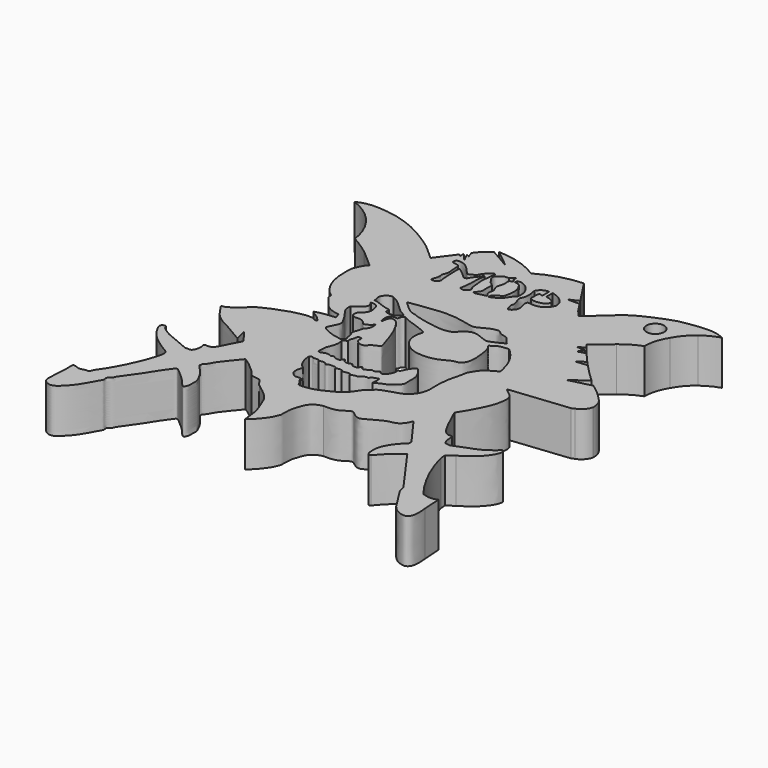
from build123d import *

# Parameters (mm, degrees)
F1_DEPTH = 5
F2_D     = 2
F2_DEPTH = 13.5
F2_TIP   = 0.600860619


with BuildPart() as f1:
    # F0 (on Top) → F1 (new body)
    with BuildSketch(Plane.XY):
        with BuildLine():
            ThreePointArc((-20.6029620022, 21.1226996034), (-17.5915636948, 19.019722507), (-16.1475036293, 15.6424865127))
            ThreePointArc((-16.1475036293, 15.6424865127), (-15.0464363703, 14.9775310986), (-13.9912227169, 14.2419775948))
            Line((-13.9912227169, 14.2419775948), (-11.9417123497, 12.4597940594))
            add(Edge.make_bspline(
                [(-12.1965548024, 7.2102304548), (-12.3502998605, 7.4831671233), (-12.5147308437, 7.918563535), (-12.7293340893, 8.6338874307), (-12.8327536648, 9.5869088664), (-12.8349054333, 10.6792935822), (-12.8027446008, 11.1125926196), (-12.2509882508, 12.2447047975), (-12.0226823195, 12.4034826204), (-11.9417123497, 12.4597940594)],
                knots=[0.8610480247, 0.8610480247, 0.8610480247, 0.8610480247, 0.8811330773, 0.9001834199, 0.9227784911, 0.945893675, 0.9616042621, 0.9863827378, 1, 1, 1, 1], degree=3))
            Line((-12.1965548024, 7.2102304548), (-11.8690758114, 6.7050356711))
            add(Edge.make_bspline(
                [(-11.6388598274, 6.4153944981), (-11.7173747261, 6.5058097894), (-11.7950645675, 6.6040888756), (-11.8690758114, 6.7050356711)],
                knots=[0.8422887794, 0.8422887794, 0.8422887794, 0.8422887794, 0.8493024804, 0.8493024804, 0.8493024804, 0.8493024804], degree=3))
            Line((-11.6388598274, 6.4153944981), (-11.4010572433, 6.1705708504))
            add(Edge.make_bspline(
                [(-8.2604521886, 3.4468797967), (-8.4593902999, 3.4581469309), (-8.8945130912, 3.5751560394), (-9.4160163716, 3.7356827733), (-9.9909022798, 4.1606108445), (-10.1208112278, 4.4103187237), (-10.540425506, 4.8665439074), (-10.7332609152, 5.1282105819), (-11.0928393262, 5.6046851275), (-10.9504645183, 5.8646077471), (-11.2233401518, 6.0114178789), (-11.4010572433, 6.1705708504)],
                knots=[0.6950364261, 0.6950364261, 0.6950364261, 0.6950364261, 0.7129994084, 0.7302227681, 0.7486757288, 0.761065719, 0.7782452685, 0.7921804993, 0.8088061225, 0.8190631278, 0.835195334, 0.835195334, 0.835195334, 0.835195334], degree=3))
            add(Edge.make_bspline(
                [(-8.04425776, 2.8521639761), (-7.9018632901, 2.858641559), (-7.7057651467, 2.8469124875), (-7.5831119329, 2.8591957281), (-7.4479762519, 2.8711507591), (-7.505413234, 3.0021417322), (-7.7961410323, 3.4541077042), (-7.9021987786, 3.4673998991), (-8.1104128522, 3.438382112), (-8.2604521886, 3.4468797967)],
                knots=[0.6221073953, 0.6221073953, 0.6221073953, 0.6221073953, 0.6354090806, 0.6434381095, 0.6504907803, 0.6579034221, 0.674423125, 0.6814887257, 0.6950364261, 0.6950364261, 0.6950364261, 0.6950364261], degree=3))
            add(Edge.make_bspline(
                [(-12.3581970111, -5.6642671116), (-12.5904511424, -5.5812313985), (-13.0193487189, -5.3035516251), (-13.6976748576, -4.9215909797), (-14.6685644807, -4.3370329977), (-15.1784801551, -4.1175978961), (-15.7822788069, -3.7457351464), (-16.4224422592, -3.1712375943), (-16.7599481469, -2.645328985), (-17.0923394133, -2.2265555734), (-17.2212769529, -2.0106109394), (-17.3896610291, -1.7573138007), (-17.1319935898, -1.7444644607), (-16.9508920629, -1.7170211764), (-16.347646044, -1.3596815627), (-15.645035849, -0.848528458), (-15.2656555451, -0.37634208), (-15.0754605235, -0.2604548851), (-14.734679896, 0.0366996912), (-14.178640127, 0.2610233151), (-13.6015369056, 0.5853071698), (-12.8447573829, 0.8220084278), (-12.1648413666, 1.1160641981), (-11.595046482, 1.272849878), (-10.9995895136, 1.4056237292), (-10.3895434203, 1.5428319889), (-9.6396418204, 1.5312353279), (-9.4289246698, 1.417578834), (-9.3011799222, 1.2945856497), (-8.942384529, 1.276901966), (-9.0026734788, 1.4242730407), (-9.167712209, 1.5846567137), (-9.5309989371, 1.9880562353), (-10.2229826163, 2.3564941518), (-10.2892403261, 2.4314994287), (-10.302815711, 2.5023911971), (-10.2349771538, 2.5157399501), (-10.1672388489, 2.5081225633), (-9.8508510482, 2.6248918916), (-9.3754645701, 2.724901108), (-8.7177845236, 2.771494927), (-8.242723901, 2.8431356698), (-8.04425776, 2.8521639761)],
                knots=[0.0199809931, 0.0199809931, 0.0199809931, 0.0199809931, 0.0393496026, 0.0597271396, 0.0835928224, 0.1005434587, 0.1193240265, 0.1403089769, 0.158438488, 0.174595577, 0.1865174997, 0.1969260736, 0.2062553482, 0.2161564821, 0.2346403213, 0.2565308226, 0.2735861318, 0.2840287475, 0.2987882298, 0.3163830901, 0.3348196829, 0.3549968985, 0.3744741565, 0.3917947559, 0.4092021997, 0.4275883294, 0.4468781727, 0.4573928431, 0.4670857793, 0.4791440786, 0.4858131114, 0.4964248036, 0.5137198846, 0.5335221874, 0.5402661667, 0.54539731, 0.5505805585, 0.5563736505, 0.5689626198, 0.5850282163, 0.603567812, 0.6221073953, 0.6221073953, 0.6221073953, 0.6221073953], degree=3))
            Line((-12.3581970111, -5.6642671116), (-12.6814246178, -4.32879664))
            Line((-12.6814246178, -4.32879664), (-11.5899201483, -5.809974391))
            add(Edge.make_bspline(
                [(-11.5899201483, -5.809974391), (-11.761671997, -6.1515096125), (-12.1023394972, -6.8289401669), (-12.5988375731, -7.7793439457), (-13.0560319176, -8.6202165569), (-14.0611028159, -8.3810100434), (-13.6893610625, -9.0087176513), (-14.0412955656, -10.064201964), (-14.4145629084, -9.9866002857), (-14.6357854762, -9.9824532437), (-14.8157372232, -10.0789508645), (-16.281058055, -9.3570080841), (-16.8233033734, -9.212552149), (-17.7368272991, -8.7952962439), (-18.6917469793, -8.1412114636), (-18.6420124904, -7.8298569891), (-18.9893398137, -7.7692027771), (-19.3106699916, -8.0342693106), (-19.0208951386, -8.680301289), (-18.5961106249, -9.4212285605), (-17.9192155256, -10.1285007663), (-16.9946139375, -10.8428939411), (-16.0873411982, -11.4169768576), (-15.5695893324, -11.6777704888), (-15.5798054281, -12.459245462), (-16.2005580806, -14.2818357649), (-17.0898354691, -16.1841050865), (-17.9990009864, -17.7647021784), (-18.4788322489, -18.2943472783), (-18.6390866322, -18.8999775429), (-19.0640131121, -18.7354536271), (-19.615346749, -19.099336736), (-20.4150388035, -18.6117409365), (-20.5369505302, -18.9048172824), (-20.4745198098, -19.3549123287), (-20.5633095325, -20.6757675795), (-20.6104330874, -21.6089482824), (-20.6526211227, -22.2395843559), (-20.5013571763, -22.6079781881), (-20.1803826553, -22.8383312321), (-19.7318715009, -23.0137189608), (-19.2193538265, -22.8744691129), (-18.7003457403, -22.3844825927), (-18.0593824453, -21.7304410154), (-17.3644822048, -20.6360646539), (-16.8172253424, -19.5595324477), (-16.5714630416, -19.2353425016), (-16.7570703992, -18.7742146415), (-16.2597684066, -18.5543558491), (-16.1987565932, -18.1739453761), (-15.4476121444, -17.1851846193), (-14.4609757351, -15.7871082425), (-13.8660241761, -14.7528565805), (-13.1529493933, -13.8016805992), (-12.8956471778, -13.4382777026), (-12.1402183108, -14.1250996886), (-11.3282640309, -14.7873756688), (-10.5542045699, -15.7471405416), (-10.4835155205, -15.8130234223), (-10.2753596318, -15.9090116166), (-10.1982709972, -15.7072660935), (-10.0523513853, -15.47296592), (-10.0750379365, -14.8415342807), (-10.0095114609, -14.292303092), (-10.5072174977, -13.352197784), (-10.9709437469, -12.6407861923), (-11.750335269, -11.9121516462), (-11.7388578236, -11.78510289), (-11.6600968913, -11.6740233806), (-11.7464815118, -11.5146223585), (-11.3969134992, -11.2917363839), (-11.0903574926, -10.5436660123), (-10.3206257246, -9.6014779347), (-9.6643011605, -8.7958952944), (-9.313037619, -8.364749141)],
                knots=[0, 0, 0, 0, 0.0179813568, 0.0356657813, 0.051329078, 0.0651099748, 0.0766372495, 0.0935148294, 0.1026170722, 0.1101464218, 0.1172045658, 0.1380930678, 0.1517065559, 0.1686436507, 0.1862776399, 0.1941540818, 0.2029227342, 0.2124825546, 0.225756734, 0.2415613643, 0.2581194594, 0.2765443366, 0.2940493854, 0.305875686, 0.3193973265, 0.3426850978, 0.3679383695, 0.3903240637, 0.4046447144, 0.416373877, 0.4260507347, 0.4393671317, 0.4542499545, 0.4614022989, 0.4726186512, 0.4920540368, 0.5088224874, 0.5218416547, 0.5320047128, 0.5423752, 0.5538059057, 0.5656121747, 0.5796000293, 0.5956835108, 0.6152465419, 0.6336595403, 0.6438739959, 0.6542959706, 0.6653348002, 0.6752500928, 0.6936720731, 0.7160143125, 0.7349445332, 0.7530770661, 0.7623269307, 0.7776086779, 0.7964830854, 0.8143398494, 0.8197448066, 0.8267371939, 0.8336105298, 0.8424634875, 0.8555147647, 0.8681538827, 0.8849009963, 0.9015710239, 0.9181986098, 0.9233461612, 0.9291090514, 0.9352376166, 0.9449772073, 0.9599565939, 0.9785688524, 1, 1, 1, 1], degree=3))
            add(Edge.make_bspline(
                [(-2.1674414165, -17.3634011298), (-2.2083754085, -17.0670616618), (-2.2889277013, -16.483907601), (-2.3687674967, -15.6105740644), (-2.5056489877, -15.180468512), (-2.7149333593, -14.5715948025), (-3.0057117915, -13.9808265561), (-3.2610484039, -13.1945992574), (-4.0167638414, -12.4073570072), (-4.8092463789, -11.8571987969), (-5.5319002932, -11.302861115), (-5.811512679, -10.4873353187), (-7.0168671674, -10.6046346662), (-7.2475569156, -9.9817356818), (-7.8224846209, -9.4881864383), (-8.3692761757, -9.0207724304), (-8.9599333798, -8.5668206068), (-9.2080848604, -8.4248106056), (-9.313037619, -8.364749141)],
                knots=[0, 0, 0, 0, 0.0689009641, 0.1355873292, 0.1841509068, 0.2409673149, 0.2997760241, 0.3648024212, 0.4395050627, 0.5112588235, 0.5792603578, 0.641576026, 0.7135666611, 0.7681324686, 0.8301936499, 0.8927655608, 0.9546464515, 1, 1, 1, 1], degree=3))
            add(Edge.make_bspline(
                [(1.6768131172, -11.058810167), (1.4498258422, -11.1119512781), (0.9778327854, -11.2224519019), (0.3269774066, -11.7855546665), (0.0646584188, -12.5740691446), (-0.1527713728, -13.1811284517), (-0.2097492346, -13.8412703608), (-0.2329829382, -14.3559228246), (-0.1924124239, -14.7284014532), (-0.3964332077, -15.1432360242), (-0.5584881611, -15.5322147196), (-0.8834596458, -15.9997141654), (-1.136769425, -16.3273670151), (-1.4494183058, -16.7034452851), (-1.7552805529, -17.0057514481), (-2.0248897803, -17.2397029532), (-2.1674414165, -17.3634011298)],
                knots=[0, 0, 0, 0, 0.0808085825, 0.1680318417, 0.255018001, 0.3325718365, 0.4106102442, 0.4794380848, 0.5373322163, 0.601038936, 0.6646014985, 0.736379439, 0.799216676, 0.8654979694, 0.928884168, 1, 1, 1, 1], degree=3))
            add(Edge.make_bspline(
                [(9.6936440095, -8.3805257455), (9.6053730454, -8.6062045499), (9.4248404792, -9.0677648615), (8.7644476462, -9.7019868071), (7.8391484374, -9.6802752734), (5.9960176715, -10.8377393732), (5.5709076534, -10.9653133541), (5.084651123, -10.8502179729), (4.5962398094, -10.4018320652), (4.31685127, -10.2638895059), (3.9607013957, -10.3984297753), (3.3525593133, -10.8740414946), (2.5884025531, -11.0445659428), (2.1036380444, -11.0617450847), (1.815664393, -11.059764931), (1.6768131172, -11.058810167)],
                knots=[0, 0, 0, 0, 0.0813790915, 0.1664372465, 0.2589445345, 0.3967526344, 0.4592648623, 0.5231293603, 0.6003716548, 0.6506866848, 0.7055950558, 0.7891929021, 0.8731143432, 0.9388199746, 1, 1, 1, 1], degree=3))
            Line((9.6936440095, -8.3805257455), (12.0183676481, -11.5794716403))
            Line((12.0183676481, -11.5794716403), (12.0183676481, -11.9077553973))
            add(Edge.make_bspline(
                [(10.380987078, -15.4800917953), (10.3387332997, -15.117733548), (10.246426762, -14.3261348663), (11.0215378886, -12.8784303298), (11.6925110223, -12.2250621944), (12.0183676481, -11.9077553973)],
                knots=[0, 0, 0, 0, 0.3027512141, 0.6613826615, 1, 1, 1, 1], degree=3))
            add(Edge.make_bspline(
                [(10.8141666278, -15.8001016825), (10.7427231899, -15.8416310013), (10.5683574389, -15.9429879778), (10.4505342148, -15.6519071454), (10.380987078, -15.4800917953)],
                knots=[0, 0, 0, 0, 0.4097332049, 1, 1, 1, 1], degree=3))
            add(Edge.make_bspline(
                [(13.1668290123, -13.602392748), (12.7702129139, -13.8888540012), (11.9451949477, -14.4847342025), (11.2007367392, -15.350526951), (10.8141666278, -15.8001016825)],
                knots=[0, 0, 0, 0, 0.4807363168, 1, 1, 1, 1], degree=3))
            Line((13.1668290123, -13.602392748), (16.9230792671, -18.8517868519))
            add(Edge.make_bspline(
                [(17.1615090221, -19.6730475873), (17.034785822, -19.4525867701), (16.9331803918, -19.186956808), (16.9230792671, -18.8517868519)],
                knots=[0, 0, 0, 0, 0.8551712949, 0.8551712949, 0.8551712949, 0.8551712949], degree=3))
            Line((17.1615090221, -19.6730475873), (18.6557825655, -22.0313183963))
            add(Edge.make_bspline(
                [(20.9009312093, -20.7379574093), (20.946669412, -21.0068443415), (21.0667752252, -22.424045845), (20.5441691625, -22.9480911155), (20.0814156096, -23.008898701), (19.1827038868, -22.6588555056), (18.8077084078, -22.2142964537), (18.6557825655, -22.0313183963)],
                knots=[0, 0, 0, 0, 0.2759456386, 0.4545875307, 0.5943096845, 0.8039768536, 1, 1, 1, 1], degree=3))
            Line((20.9009312093, -20.7379574093), (20.7737311721, -18.7153462321))
            add(Edge.make_bspline(
                [(19.0693489557, -18.7153462321), (19.3211115884, -18.7936733033), (19.916140688, -18.9445847276), (20.3488546888, -18.8852960675), (20.7737311721, -18.7153462321)],
                knots=[0, 0, 0, 0, 0.4817386314, 1, 1, 1, 1], degree=3))
            ThreePointArc((19.0693489557, -18.7153462321), (17.1945449581, -15.6929535506), (15.9742087126, -12.3522160575))
            Line((15.9742087126, -12.3522160575), (15.9212257713, -11.7296464741))
            Line((15.9212257713, -11.7296464741), (16.7331937701, -11.1593846232))
            add(Edge.make_bspline(
                [(19.5059552789, -8.0829588094), (19.4447040558, -8.5108317435), (19.076332208, -9.2460772627), (17.9914928687, -10.3808130068), (17.1422320797, -10.9105939373), (16.7331937701, -11.1593846232)],
                knots=[0, 0, 0, 0, 0.310219277, 0.6584804582, 1, 1, 1, 1], degree=3))
            ThreePointArc((19.5059552789, -8.0829588094), (19.2350807313, -7.7977856695), (18.9642061838, -8.0829588094))
            add(Edge.make_bspline(
                [(15.0774473823, -9.967437324), (16.5505504071, -9.4062854741), (17.5287417336, -9.0468549853), (18.2133857161, -8.660803549), (18.9642061838, -8.0829588094)],
                knots=[0, 0, 0, 0, 0.5565007534, 1, 1, 1, 1], degree=3))
            Line((15.0774473823, -9.967437324), (14.5304155103, -9.8842515916))
            add(Edge.make_bspline(
                [(11.4801516756, -4.8446576111), (12.2792130652, -6.6117397342), (13.2242516061, -8.8699425893), (14.4148425893, -8.2242481179), (14.1074610189, -9.4350335972), (14.5304155103, -9.8842515916)],
                knots=[0, 0, 0, 0, 0.5155027122, 0.7007845535, 1, 1, 1, 1], degree=3))
            add(Edge.make_bspline(
                [(12.2916540131, 1.5507938806), (12.7276787534, 1.0922398651), (13.6267942877, 0.793434585), (13.4155968414, -1.2858010843), (12.7945104614, -2.7060380671), (11.4801516756, -4.8446576111)],
                knots=[0, 0, 0, 0, 0.2667013683, 0.5335681874, 1, 1, 1, 1], degree=3))
            Line((12.2916540131, 1.5507938806), (18.9940966666, 2.2610761225))
            Line((18.9940966666, 2.2610761225), (19.305286929, 2.4047526531))
            ThreePointArc((19.305286929, 2.4047526531), (20.0097990037, 2.8651506455), (20.4079579562, 3.6066174507))
            ThreePointArc((20.4079579562, 3.6066174507), (20.3193874403, 4.3080407583), (19.9958346784, 4.9366527237))
            ThreePointArc((19.9958346784, 4.9366527237), (18.9806691644, 5.9619052319), (17.8415514529, 6.8474076688))
            Line((17.8415514529, 6.8474076688), (15.2579825372, 6.2031652778))
            Line((15.2579825372, 6.2031652778), (17.1197786733, 7.4977375506))
            ThreePointArc((17.1197786733, 7.4977375506), (16.0491412163, 8.5243825489), (15.0177698901, 9.5904677728))
            Line((15.0177698901, 9.5904677728), (13.6827398092, 9.4481641427))
            Line((13.6827398092, 9.4481641427), (14.5777972838, 10.0705290551))
            ThreePointArc((14.5777972838, 10.0705290551), (14.0339347858, 10.6866031408), (13.5029950802, 11.3138484875))
            Line((13.5029950802, 11.3138484875), (12.5840436667, 11.0233156011))
            Line((12.5840436667, 11.0233156011), (13.0566162989, 11.6376606748))
            Line((13.0566162989, 11.6376606748), (12.4895293266, 11.4643834531))
            Line((12.4895293266, 11.4643834531), (12.8675876185, 11.763679795))
            Line((12.8675876185, 11.763679795), (12.0799662545, 11.7006702349))
            Line((12.0799662545, 11.7006702349), (12.8092804911, 12.1751222925))
            ThreePointArc((12.8092804911, 12.1751222925), (12.6443146642, 12.3873848258), (12.4807959896, 12.6007641829))
            Line((12.4807959896, 12.6007641829), (14.5000191405, 14.3246697262))
            ThreePointArc((14.5000191405, 14.3246697262), (15.5107148946, 15.0425023951), (16.6326500475, 15.5698079616))
            ThreePointArc((16.6326500475, 15.5698079616), (16.8245383582, 16.9374935756), (17.400925979, 18.1925483048))
            ThreePointArc((17.400925979, 18.1925483048), (18.1163270549, 19.25582228), (19.0566964447, 20.1264861971))
            ThreePointArc((19.0566964448, 20.1264861971), (19.9676202839, 20.6998781196), (20.9641419351, 21.1067013443))
            ThreePointArc((20.9641419351, 21.1067013443), (20.0622769035, 21.4273714063), (19.1106745535, 21.5305353114))
            ThreePointArc((19.1106745535, 21.5305353114), (17.494918218, 21.3939271519), (15.8990386297, 21.1067013443))
            ThreePointArc((15.8990386297, 21.1067013443), (14.2592549209, 20.5084373442), (12.6720489934, 19.7820849716))
            ThreePointArc((12.6720489934, 19.7820849716), (11.8479697713, 19.298407767), (11.0957566649, 18.7091492116))
            Line((11.0957566649, 18.7091492116), (8.5127558559, 16.3910705596))
            Line((8.5127558559, 16.3910705596), (7.823956199, 17.2255784273))
            Line((7.823956199, 17.2255784273), (7.1296900244, 18.291907385))
            Line((7.1296900244, 18.291907385), (5.743692629, 18.291907385))
            Line((5.743692629, 18.291907385), (6.8139770912, 18.7768133983))
            Line((6.8139770912, 18.7768133983), (4.9760327674, 21.5997267514))
            ThreePointArc((4.9760327674, 21.5997267514), (2.470754193, 21.1792888514), (0.1411859703, 20.1662238687))
            ThreePointArc((0.1411859703, 20.1662238687), (-2.1388945551, 21.2114676219), (-4.6169091947, 21.5997267514))
            Line((-4.6169091947, 21.5997267514), (-2.5629734155, 19.9449639767))
            Line((-2.5629734155, 19.9449639767), (-4.9981252836, 21.3476927034))
            ThreePointArc((-4.9981252836, 21.3476927034), (-5.7618963683, 20.7054799466), (-6.4152670093, 19.9512317777))
            Line((-6.4152670093, 19.9512317777), (-6.1913165264, 19.281739369))
            Line((-6.1913165264, 19.281739369), (-6.5142409876, 19.3998813629))
            Line((-6.5142409876, 19.3998813629), (-6.0180397704, 18.4389837086))
            Line((-6.0180397704, 18.4389837086), (-6.8394649689, 19.3754563593))
            Line((-6.8394649689, 19.3754563593), (-6.8394649689, 18.8564229756))
            Line((-6.8394649689, 18.8564229756), (-7.0873237208, 19.0390309396))
            Line((-7.0873237208, 19.0390309396), (-8.6397584528, 16.9318690896))
            Line((-8.6397584528, 16.9318690896), (-10.2622583508, 18.3810908347))
            ThreePointArc((-10.2622583508, 18.3810908347), (-11.3785350691, 19.1686702966), (-12.5463595614, 19.8775716126))
            ThreePointArc((-12.5463595614, 19.8775716126), (-15.3498488558, 21.1074830333), (-18.3747559786, 21.5788334608))
            ThreePointArc((-18.3747559786, 21.5788334608), (-19.5171424452, 21.488930721), (-20.6029620022, 21.1226996034))
        make_face()
        with BuildLine():
            add(Edge.make_bspline(
                [(-6.5327608027, 17.5191853195), (-6.3748484418, 17.4234895456), (-5.6365651898, 17.4708052331), (-5.7990185334, 16.6081123486), (-5.5555387858, 15.7371018682), (-5.8669215309, 15.1764552056), (-5.8708151654, 14.9237481), (-5.7527401438, 14.5870300173), (-6.0718190484, 13.895355508), (-5.9662190963, 13.6971696288), (-5.4300433536, 13.7072170087), (-5.1873519927, 14.1436105181), (-5.3159272554, 14.3295967542), (-5.4181501645, 16.7450430853), (-5.3160856513, 16.9213788182), (-5.0990932249, 16.7504733804), (-4.7109284165, 16.4879298969), (-4.266704401, 16.0589203452), (-4.0377927519, 15.834100095), (-3.897375245, 15.8351288787), (-3.6878984093, 15.8535489132), (-3.5789232755, 16.1506190902), (-3.351938068, 16.4713045175), (-3.005734269, 16.8250021688), (-2.6440367711, 17.5329001114), (-2.8894746827, 16.0651132518), (-2.7875019448, 15.6050809447), (-2.9408976883, 14.2824267235), (-3.0722308887, 14.0475795423), (-2.6172554539, 13.9408469698), (-2.3923457368, 14.0585021081), (-1.980889262, 14.403116041), (-2.128946951, 14.6708063351), (-2.2514500178, 14.7184476404), (-2.2831222674, 15.1756058931), (-2.3295033655, 15.7507585172), (-2.425786598, 16.4138654632), (-2.3185863377, 17.0435299004), (-2.2786610411, 17.6286883894), (-2.135973059, 18.0475221391), (-2.4457532459, 18.1612584596), (-2.6507968129, 17.9255590236), (-3.177116447, 17.4678914379), (-3.3910902868, 16.8922437211), (-3.7344724565, 16.7994067453), (-4.1526126676, 16.4796251985), (-4.3890724961, 16.7745451418), (-4.7896158566, 17.1992804798), (-5.253486026, 17.7242731105), (-5.8784213159, 18.0356818537), (-6.5008772214, 18.0579147394), (-6.6597312966, 17.7844870874), (-6.6300710597, 17.5781558796), (-6.5327608027, 17.5191853195)],
                knots=[0, 0, 0, 0, 0.0246614949, 0.0485994997, 0.0767657835, 0.0990043667, 0.112854626, 0.130009994, 0.1548053205, 0.1664415199, 0.1863172472, 0.2048211466, 0.2199223707, 0.2649403173, 0.275151451, 0.2885440667, 0.309127104, 0.3324121137, 0.3482472655, 0.3586111661, 0.3709359946, 0.3864988063, 0.4046846859, 0.4267734987, 0.4447663178, 0.4738739773, 0.4982401656, 0.5307988884, 0.5434648015, 0.5608947357, 0.576466356, 0.5964929476, 0.6104899015, 0.6201958353, 0.6387398738, 0.6615799777, 0.6852757645, 0.7085607671, 0.7313034222, 0.749029496, 0.7625180384, 0.7779617692, 0.8025220407, 0.8246108686, 0.8417132472, 0.8610901392, 0.8768322806, 0.8992944111, 0.9237530004, 0.9482244378, 0.9699730011, 0.984802859, 1, 1, 1, 1], degree=3))
        make_face(mode=Mode.SUBTRACT)
        with BuildLine():
            add(Edge.make_bspline(
                [(-0.8483318961, 18.2840451598), (-1.0114835564, 18.2072715981), (-1.2634396973, 18.3115930841), (-1.7003885983, 17.9564807232), (-2.0807745461, 17.7561257957), (-2.0353868889, 17.1766447957), (-1.7423416676, 16.8596623118), (-1.4758024298, 16.4449185041), (-1.3718480477, 16.4350308478)],
                knots=[0, 0, 0, 0, 0.0267141766, 0.0564116804, 0.0826888888, 0.111361588, 0.1403955551, 0.1702693254, 0.1702693254, 0.1702693254, 0.1702693254], degree=3))
            add(Edge.make_bspline(
                [(-0.1690216065, 18.1514766594), (-0.2281947297, 18.149664051), (-0.4091389205, 18.2030109456), (-0.1803598606, 18.8772600194), (-0.648952205, 18.3778663872), (-0.8483318961, 18.2840451598)],
                knots=[0.9244373769, 0.9244373769, 0.9244373769, 0.9244373769, 0.9422389396, 0.967353907, 1, 1, 1, 1], degree=3))
            add(Edge.make_bspline(
                [(0.0943494252, 18.2405747631), (0.0594572467, 18.2292988279), (-0.050911535, 18.1881064671), (-0.1109887882, 18.1532543377), (-0.1690216065, 18.1514766594)],
                knots=[0.8999068914, 0.8999068914, 0.8999068914, 0.8999068914, 0.9069788618, 0.9244373769, 0.9244373769, 0.9244373769, 0.9244373769], degree=3))
            add(Edge.make_bspline(
                [(0, 14.3471976528), (0.0673188304, 14.3524413667), (0.4051495367, 14.4051046128), (1.1215237724, 14.9291264779), (1.4125637475, 15.2874755457), (1.742939517, 15.9282948112), (2.0027801262, 15.9160389572), (2.0835342171, 17.0628713023), (1.3599196421, 17.8747628531), (0.9984012943, 18.1188567537), (0.5252213674, 18.3442921296), (0.2002409824, 18.2747952214), (0.0943494252, 18.2405747631)],
                knots=[0.6026736293, 0.6026736293, 0.6026736293, 0.6026736293, 0.6134119734, 0.6553723204, 0.6857472435, 0.7189536726, 0.7363381198, 0.7773520526, 0.8204884436, 0.8479338347, 0.8784447188, 0.8999068914, 0.8999068914, 0.8999068914, 0.8999068914], degree=3))
            add(Edge.make_bspline(
                [(-0.2691223056, 14.3409602613), (-0.1768663373, 14.3429714768), (-0.0897855361, 14.3402039238), (0, 14.3471976528)],
                knots=[0.5883515151, 0.5883515151, 0.5883515151, 0.5883515151, 0.6026736293, 0.6026736293, 0.6026736293, 0.6026736293], degree=3))
            add(Edge.make_bspline(
                [(-1.094278679, 16.1960963374), (-1.0976910261, 16.1555249115), (-1.1256042641, 15.8331140363), (-1.1807006416, 15.4442098382), (-1.0712037955, 14.7061391184), (-1.5455829554, 14.323414837), (-1.6142727098, 14.1290140137), (-1.2513998767, 14.090673029), (-0.637906092, 14.3239721147), (-0.3225680006, 14.3397951246), (-0.2691223056, 14.3409602613)],
                knots=[0.4007773831, 0.4007773831, 0.4007773831, 0.4007773831, 0.4054876422, 0.4393902462, 0.4735729976, 0.5046742959, 0.5194369016, 0.5409382195, 0.580054433, 0.5883515151, 0.5883515151, 0.5883515151, 0.5883515151], degree=3))
            Line((-1.094278679, 16.1960963374), (-1.3718480477, 16.4350308478))
        make_face(mode=Mode.SUBTRACT)
        with BuildLine():
            add(Edge.make_bspline(
                [(-8.3830459043, 5.3127408028), (-8.3940597447, 5.0777512633), (-8.4158385536, 4.6130820755), (-8.0395670438, 4.0638324237), (-7.5004379381, 3.4007418352), (-7.2507926236, 2.7889510474), (-6.8583607581, 2.3470451893), (-7.2475506238, 1.5400259231), (-7.4311082064, 1.1710155962), (-7.684005163, 0.7224976126), (-6.8822248872, 0.3319713145), (-6.0490013419, -0.0093856315), (-5.3952506303, -0.0624924128), (-5.2036927412, -0.1279320912)],
                knots=[0, 0, 0, 0, 0.023441613, 0.0463535326, 0.0727577908, 0.0959584121, 0.1165068076, 0.1421194096, 0.1614897362, 0.1787994952, 0.2031084384, 0.2336416731, 0.251372947, 0.251372947, 0.251372947, 0.251372947], degree=3))
            add(Edge.make_bspline(
                [(-7.4273948558, 6.9859479554), (-7.4050513485, 6.9091412079), (-7.2692398671, 6.7231148531), (-7.1697119763, 6.4673261331), (-7.2173907018, 6.2081272216), (-7.7469279046, 5.6951530579), (-8.1677574672, 5.442164804), (-8.3830459043, 5.3127408028)],
                knots=[0.9075821697, 0.9075821697, 0.9075821697, 0.9075821697, 0.923136823, 0.9377895399, 0.951406795, 0.9751406363, 1, 1, 1, 1], degree=3))
            add(Edge.make_bspline(
                [(-7.4288295582, 7.5301378965), (-7.4101794187, 7.3994676083), (-7.4189345818, 7.1603721722), (-7.444267123, 7.0439470851), (-7.4273948558, 6.9859479554)],
                knots=[0.8785937792, 0.8785937792, 0.8785937792, 0.8785937792, 0.8958363741, 0.9075821697, 0.9075821697, 0.9075821697, 0.9075821697], degree=3))
            add(Edge.make_bspline(
                [(-6.5555996262, 9.0675801039), (-6.7805151147, 9.0666037069), (-7.0482609087, 9.018530442), (-7.2716290979, 8.7703414066), (-7.5694057781, 8.5458795402), (-7.5529740469, 7.9465680518), (-7.4492660034, 7.673323752), (-7.4288295582, 7.5301378965)],
                knots=[0.7865357045, 0.7865357045, 0.7865357045, 0.7865357045, 0.8064943004, 0.8220711192, 0.838672488, 0.8596996928, 0.8785937792, 0.8785937792, 0.8785937792, 0.8785937792], degree=3))
            add(Edge.make_bspline(
                [(-4.9596737231, 9.0362414759), (-5.0346964758, 9.026680953), (-5.4893617317, 8.9853427411), (-6.184400489, 9.0691915434), (-6.5555996262, 9.0675801039)],
                knots=[0.7466653621, 0.7466653621, 0.7466653621, 0.7466653621, 0.7535961607, 0.7865357045, 0.7865357045, 0.7865357045, 0.7865357045], degree=3))
            add(Edge.make_bspline(
                [(6.8161031231, 8.4036868566), (6.7660423749, 8.4507670515), (6.5092237632, 8.7019243916), (6.2990413394, 9.0209926075), (6.1006905489, 9.2346374411), (5.9076129278, 9.3473798961), (5.3350842251, 9.3863535327), (4.9687300084, 9.7555885312), (4.7697635111, 9.8542130617), (4.3532575424, 9.8137746211), (3.717592733, 9.6185130483), (2.7930037396, 9.0266055369), (2.195318318, 9.0002462485), (1.3775317202, 9.2496336959), (0.8115180032, 9.331030783), (0.3379642291, 9.4559696578), (-1.4151669229, 9.5732427099), (-2.988925361, 9.2454234154), (-4.2776208076, 9.1821946498), (-4.7532296561, 9.062549671), (-4.9596737231, 9.0362414759)],
                knots=[0.3536083579, 0.3536083579, 0.3536083579, 0.3536083579, 0.3586701658, 0.381299825, 0.3956764223, 0.4086196281, 0.4297653997, 0.4498459333, 0.4626646007, 0.4800084793, 0.5035730736, 0.5328679813, 0.5546631536, 0.5805981384, 0.6016341725, 0.6210827981, 0.6579116053, 0.6951431805, 0.7275935178, 0.7466653621, 0.7466653621, 0.7466653621, 0.7466653621], degree=3))
            add(Edge.make_bspline(
                [(7.6669156083, 7.6605655853), (7.3739983276, 7.9202820595), (7.0585166009, 8.1757063687), (6.8161031231, 8.4036868566)],
                knots=[0.3290971289, 0.3290971289, 0.3290971289, 0.3290971289, 0.3536083579, 0.3536083579, 0.3536083579, 0.3536083579], degree=3))
            add(Edge.make_bspline(
                [(7.0084095933, -2.2698552348), (7.0007780714, -1.9680162605), (6.9840913533, -1.3080296946), (7.1254872011, -0.0001355957), (7.4994574307, 1.1400460625), (7.5492172412, 1.7810783393), (7.6725394429, 1.9625468715), (8.0860563781, 2.696789682), (8.5682114362, 3.2349954401), (9.7104571973, 3.7808581734), (9.7148676604, 3.8646708704), (9.7162466545, 4.0557934065), (9.3922631373, 5.295283035), (8.8289144398, 6.4022322861), (8.2146647755, 7.164170137), (7.7460991889, 7.590357094), (7.6669156083, 7.6605655853)],
                knots=[0, 0, 0, 0, 0.0275211537, 0.0601764293, 0.0917158206, 0.1131814168, 0.1261939158, 0.1509884724, 0.1774871114, 0.2078708058, 0.2142759641, 0.2252416045, 0.2566151127, 0.2890538304, 0.3224710709, 0.3290971289, 0.3290971289, 0.3290971289, 0.3290971289], degree=3))
            add(Edge.make_bspline(
                [(-5.2719065552, -4.4326283936), (-5.2694280057, -4.4760036259), (-5.2295917519, -5.0499728211), (-5.0042653701, -5.7929796239), (-4.584308701, -6.2807569893), (-4.250405592, -6.4902502234), (-4.4867170032, -6.9609762131), (-4.4922767041, -7.3208012868), (-4.4938205901, -7.7532805124), (-4.0510933786, -8.0485035317), (-3.9096932916, -8.2609558976), (-3.2353810253, -8.1062796601), (-3.1660171698, -8.3621899103), (-2.967384696, -8.695796468), (-2.6875593963, -9.0074956138), (-2.633822457, -9.355993789), (-1.443692626, -9.2480281644), (-0.3803327068, -8.9113127916), (0.6979700159, -8.318088912), (1.6991544658, -7.8289373821), (2.3540846796, -6.5375853895), (3.0076257032, -6.100711019), (3.4417025406, -5.5628444168), (4.3590767989, -5.3324783993), (5.0694764634, -5.0757339648), (5.6968558715, -4.8873532932), (6.3036829988, -4.4666146925), (6.7790748491, -3.8153146019), (7.0517430144, -2.9361750442), (7.0220689383, -2.4798892438), (7.0084095933, -2.2698552348)],
                knots=[0.3747381686, 0.3747381686, 0.3747381686, 0.3747381686, 0.3773536376, 0.4097649423, 0.431919453, 0.4478383689, 0.4668780118, 0.4844549467, 0.502435188, 0.5223284306, 0.5364167255, 0.5581855123, 0.5710198413, 0.5889120762, 0.6073609474, 0.6217085394, 0.6506547727, 0.6821255989, 0.7133294367, 0.7433450056, 0.7769024577, 0.8019215827, 0.8249321439, 0.8522730567, 0.8773046874, 0.9001289783, 0.9242066778, 0.9498221723, 0.976902524, 1, 1, 1, 1], degree=3))
            add(Edge.make_bspline(
                [(-5.2454476754, -3.0644561969), (-5.2692694906, -3.4648347915), (-5.2979301957, -3.9772082103), (-5.2719065552, -4.4326283936)],
                knots=[0.347276935, 0.347276935, 0.347276935, 0.347276935, 0.3747381686, 0.3747381686, 0.3747381686, 0.3747381686], degree=3))
            add(Edge.make_bspline(
                [(-4.9262600951, -0.3084103519), (-4.7361400411, -0.5549805721), (-4.8429996508, -1.473731228), (-5.2196977482, -2.1671825805), (-5.2138380165, -2.5434839511), (-5.2380805149, -2.9406346774), (-5.2454476754, -3.0644561969)],
                knots=[0.2619340345, 0.2619340345, 0.2619340345, 0.2619340345, 0.2921329314, 0.3174574982, 0.338784244, 0.347276935, 0.347276935, 0.347276935, 0.347276935], degree=3))
            add(Edge.make_bspline(
                [(-5.2036927412, -0.1279320912), (-5.089597181, -0.1669092213), (-4.9927484353, -0.2221803917), (-4.9262600951, -0.3084103519)],
                knots=[0.251372947, 0.251372947, 0.251372947, 0.251372947, 0.2619340345, 0.2619340345, 0.2619340345, 0.2619340345], degree=3))
        make_face(mode=Mode.SUBTRACT)
        with BuildLine():
            add(Edge.make_bspline(
                [(2.464838542, 17.7272399876), (2.4244064792, 17.5440519408), (2.6304765231, 17.2079944074), (2.548484494, 16.1863323241), (2.3565900343, 15.9391444482), (2.3172415344, 15.6220667178), (2.4508429081, 15.3213917896), (2.7234882288, 14.6340462549), (2.4972221758, 14.2635238843), (2.6538520767, 14.1058349889), (2.7056716338, 13.3202939329), (3.4198853834, 13.85079943), (3.5578998579, 14.3967471492), (3.3700287652, 14.8908671403), (3.2413094209, 15.7135498736), (3.8056542076, 15.5551472105), (4.4879992676, 15.5915631108), (5.1202359353, 15.7945598109), (6.0355063672, 16.7973858588), (5.2476476249, 17.9704762287), (4.3273655072, 18.358435961), (3.9791150722, 18.4232501125)],
                knots=[0, 0, 0, 0, 0.046848488, 0.1085084057, 0.1434452499, 0.1761286253, 0.2126975848, 0.2657660495, 0.3031805018, 0.3315391388, 0.3778580376, 0.426161914, 0.4727038228, 0.5198547314, 0.5697285081, 0.6092860173, 0.6614637571, 0.7127258162, 0.7785833034, 0.8532626596, 0.9001831293, 0.9001831293, 0.9001831293, 0.9001831293], degree=3))
            add(Edge.make_bspline(
                [(3.5716684069, 18.4584685393), (3.4368549653, 18.4555296012), (2.8859371808, 18.3752004059), (2.5184643317, 17.9702056681), (2.464838542, 17.7272399876)],
                knots=[0.9188180789, 0.9188180789, 0.9188180789, 0.9188180789, 0.9378639875, 1, 1, 1, 1], degree=3))
            add(Edge.make_bspline(
                [(3.9791150722, 18.4232501125), (3.8408038122, 18.4489917226), (3.70357294, 18.4613440631), (3.5716684069, 18.4584685393)],
                knots=[0.9001831293, 0.9001831293, 0.9001831293, 0.9001831293, 0.9188180789, 0.9188180789, 0.9188180789, 0.9188180789], degree=3))
        make_face(mode=Mode.SUBTRACT)
        with BuildLine():
            add(Edge.make_bspline(
                [(-8.04425776, 2.8521639761), (-7.9018632901, 2.858641559), (-7.7057651467, 2.8469124875), (-7.5831119329, 2.8591957281), (-7.4479762519, 2.8711507591), (-7.505413234, 3.0021417322), (-7.7961410323, 3.4541077042), (-7.9021987786, 3.4673998991), (-8.1104128522, 3.438382112), (-8.2604521886, 3.4468797967)],
                knots=[0.6221073953, 0.6221073953, 0.6221073953, 0.6221073953, 0.6354090806, 0.6434381095, 0.6504907803, 0.6579034221, 0.674423125, 0.6814887257, 0.6950364261, 0.6950364261, 0.6950364261, 0.6950364261], degree=3))
            Line((-8.2604521886, 3.4468797967), (-8.04425776, 2.8521639761))
        make_face()
        with BuildLine():
            Line((-4.7277102406, 0.2033870907), (-5.2036927412, -0.1279320912))
            add(Edge.make_bspline(
                [(-5.2036927412, -0.1279320912), (-5.089597181, -0.1669092213), (-4.9927484353, -0.2221803917), (-4.9262600951, -0.3084103519)],
                knots=[0.251372947, 0.251372947, 0.251372947, 0.251372947, 0.2619340345, 0.2619340345, 0.2619340345, 0.2619340345], degree=3))
            Line((-4.9262600951, -0.3084103519), (-4.4398466125, 0))
            add(Edge.make_bspline(
                [(-4.7277102406, 0.2033870907), (-4.6182205093, 0.0784984236), (-4.4834449654, -0.0195435779), (-4.4398466125, 0)],
                knots=[0.3958192568, 0.3958192568, 0.3958192568, 0.3958192568, 0.4083769019, 0.4083769019, 0.4083769019, 0.4083769019], degree=3))
        make_face()
        with BuildLine():
            add(Edge.make_bspline(
                [(-7.4288295582, 7.5301378965), (-7.4101794187, 7.3994676083), (-7.4189345818, 7.1603721722), (-7.444267123, 7.0439470851), (-7.4273948558, 6.9859479554)],
                knots=[0.8785937792, 0.8785937792, 0.8785937792, 0.8785937792, 0.8958363741, 0.9075821697, 0.9075821697, 0.9075821697, 0.9075821697], degree=3))
            add(Edge.make_bspline(
                [(-7.4273948558, 6.9859479554), (-7.3195412175, 6.9959931812), (-7.0914370851, 7.0172382457), (-6.6484825155, 6.8544551545), (-6.553884648, 6.5696500525), (-6.3358297768, 5.9037635119), (-6.5197957152, 5.3550810482), (-6.8161128439, 5.0187534553), (-7.0924191227, 4.8615839869), (-7.2474163615, 4.5517212214), (-7.214523074, 4.028215255), (-6.6789253388, 3.8935347404), (-6.2557042919, 3.9640164822), (-5.8086411855, 3.8163008114), (-5.5345924654, 3.5387778774), (-5.3585189773, 3.304863014), (-5.1134514952, 3.5399199026), (-4.7037834883, 3.5237546813), (-4.4416467742, 4.2086229244), (-4.4478023195, 3.7634351496), (-4.3818366932, 3.3319620027), (-4.5421574147, 2.9612228275), (-4.8522509945, 2.7247280476), (-4.941787787, 2.1251736993), (-5.2530104035, 1.5482805445), (-4.8420749148, 0.8988762374), (-4.9522019924, 0.500504385), (-4.7721982387, 0.2541320028), (-4.7277102406, 0.2033870907)],
                knots=[0, 0, 0, 0, 0.0140360627, 0.0296935187, 0.0425493249, 0.0623201533, 0.080461242, 0.0962491989, 0.1094595246, 0.1232796733, 0.1393544095, 0.1558861692, 0.1718352519, 0.1879149621, 0.2031339351, 0.2144969766, 0.2267599171, 0.2421288474, 0.2587015523, 0.2700363608, 0.2868224972, 0.3015174756, 0.3159904817, 0.334354561, 0.3532849414, 0.3730363077, 0.3907168194, 0.3958192568, 0.3958192568, 0.3958192568, 0.3958192568], degree=3))
            add(Edge.make_bspline(
                [(-4.7277102406, 0.2033870907), (-4.6182205093, 0.0784984236), (-4.4834449654, -0.0195435779), (-4.4398466125, 0)],
                knots=[0.3958192568, 0.3958192568, 0.3958192568, 0.3958192568, 0.4083769019, 0.4083769019, 0.4083769019, 0.4083769019], degree=3))
            add(Edge.make_bspline(
                [(-4.4398466125, 0), (-4.398037899, 0.0187413468), (-4.4927456194, 0.3045798634), (-4.2973260261, 0.5965818863), (-4.2434715009, 1.1540411819), (-4.04722981, 1.2062878748), (-3.6675613474, 1.1239498372), (-3.8513728803, 0.7226526203), (-3.682256104, 0.5145200662), (-3.4337506029, 0.2392118626), (-3.0731487346, 0.1575232146), (-2.7834011332, 0.2182917738), (-2.6379383528, 0.3110170615), (-2.3831262324, 0.6594762536), (-1.7881635738, 0.9230986121), (-1.5652058315, 0.9702845788), (-1.4808602713, 1.170345275), (-1.5648682528, 1.4321507421), (-2.1836096177, 3.4611405892), (-2.7956562201, 4.7105264031), (-3.3806543896, 5.549011904), (-3.7072336963, 5.6897439714), (-4.0610541671, 5.8287477884), (-4.3159362688, 5.5212596026), (-4.4024467894, 5.1036481143), (-4.4418271562, 4.780370206), (-4.5406251328, 4.8429934705), (-4.5887759955, 5.2013232325), (-4.6206319365, 5.3927688644), (-4.6159398569, 5.6736346285), (-4.3994630536, 6.0454039146), (-4.0626705739, 6.1246079822), (-3.6720300571, 6.0228581926), (-3.6506010633, 6.2993642791), (-3.5674970071, 6.5503755069), (-3.445330669, 6.6183424316), (-3.3235193696, 6.7304051481)],
                knots=[0.4083769019, 0.4083769019, 0.4083769019, 0.4083769019, 0.4204190768, 0.435507603, 0.4526241136, 0.4625158276, 0.4754395014, 0.4893371564, 0.5013222602, 0.5157841796, 0.5302543789, 0.5429548778, 0.552545302, 0.5681692663, 0.5876080202, 0.5987465199, 0.6085188316, 0.620494941, 0.6549404467, 0.6851788768, 0.7082520354, 0.7223747637, 0.7359870245, 0.7498692727, 0.7664010378, 0.7786415273, 0.7841903231, 0.7984637743, 0.8095624536, 0.8219539425, 0.8371449439, 0.8511674162, 0.8649174775, 0.8759352421, 0.8877021404, 0.9012484887, 0.9012484887, 0.9012484887, 0.9012484887], degree=3))
            add(Edge.make_bspline(
                [(-3.3235193696, 6.7304051481), (-3.1090672784, 6.9276945951), (-2.7197000286, 7.3595828041), (-2.7464483865, 7.5301378965)],
                knots=[0.9012484887, 0.9012484887, 0.9012484887, 0.9012484887, 0.9250972017, 0.9250972017, 0.9250972017, 0.9250972017], degree=3))
            add(Edge.make_bspline(
                [(-2.7464483865, 7.5301378965), (-2.7664538643, 7.6576984796), (-3.4009843387, 7.6109495624), (-4.2986151557, 8.3561431488), (-4.8530531341, 8.8997471973), (-4.935112038, 9.0023003595), (-4.9596737231, 9.0362414759)],
                knots=[0.9250972017, 0.9250972017, 0.9250972017, 0.9250972017, 0.9429339939, 0.9698729596, 0.9907418413, 1, 1, 1, 1], degree=3))
            add(Edge.make_bspline(
                [(-4.9596737231, 9.0362414759), (-5.0346964758, 9.026680953), (-5.4893617317, 8.9853427411), (-6.184400489, 9.0691915434), (-6.5555996262, 9.0675801039)],
                knots=[0.7466653621, 0.7466653621, 0.7466653621, 0.7466653621, 0.7535961607, 0.7865357045, 0.7865357045, 0.7865357045, 0.7865357045], degree=3))
            add(Edge.make_bspline(
                [(-6.5555996262, 9.0675801039), (-6.3886344663, 8.9921003404), (-6.0071569635, 8.8196462087), (-5.2505876757, 8.2044023623), (-4.7128646526, 7.6946527631), (-4.3230188875, 7.2578593545), (-3.4641369776, 6.8945179421), (-3.9000571646, 6.6600461632), (-4.3100609603, 6.3044660602), (-4.8365605136, 6.3084883274), (-5.3968892377, 6.3826199713), (-5.205933557, 6.992573562), (-5.6543906545, 6.9695414172), (-6.4445136724, 7.2253409786), (-7.0321999586, 7.4705036867), (-7.3089114737, 7.5121079254), (-7.4288295582, 7.5301378965)],
                knots=[0, 0, 0, 0, 0.0731862116, 0.1672138862, 0.2488055448, 0.3253657824, 0.4051584311, 0.456357354, 0.5275131737, 0.5972742542, 0.6602969366, 0.7224278359, 0.7757280666, 0.864348816, 0.941213035, 1, 1, 1, 1], degree=3))
        make_face()
        with BuildLine():
            add(Edge.make_bspline(
                [(-5.2454476754, -3.0644561969), (-5.2082459121, -3.1494364651), (-5.1116746823, -3.3696093017), (-4.5081214795, -2.9767055729), (-4.0273865937, -3.0681648725), (-3.7894227457, -3.2392947886), (-3.5291095108, -3.0146790286), (-3.4065205791, -3.1998819903), (-3.1767326794, -3.2842619509), (-2.6957934125, -3.4034593703), (-2.5006687117, -2.8832851558), (-2.3331176748, -3.024406616), (-2.2080475303, -3.3212213366), (-1.7512749717, -3.4006682831), (-1.3844333994, -3.1550080528), (-1.2468838383, -3.2876693196), (-1.1746445983, -3.4753416463), (-0.8642162403, -3.508464399), (-0.5218909782, -3.4772366443), (-0.3440470109, -3.0120431971), (-0.2174252421, -3.2436877676), (-0.0306610134, -3.5519290038), (0.7412563166, -2.9974676417), (0.7995070992, -3.0405243881), (1.082750272, -3.1306344085), (1.4632720956, -2.7373716269), (1.5494433495, -2.8826090488), (1.6768257483, -2.9991099185), (2.0680301122, -3.080729388), (2.4884048771, -2.390177128), (2.6121393264, -2.0044773943), (2.5226959526, -1.5938100146), (2.6800886187, -1.6512637194), (2.7874978004, -1.5721195269), (2.9313876041, -1.3231190932), (2.9612820816, -1.1137620124), (3.2382892108, -0.7089072289), (3.5936006038, -0.2243926131), (3.8207572457, -0.4088027874), (4.1470566991, -0.7819535914), (4.6802558559, -1.655940524), (4.5436229909, -2.7341228708), (4.6786555423, -3.3254404613), (4.2189539654, -3.7738899408), (3.4868348422, -4.4229206331), (2.8327586948, -4.5024766766), (2.2388324685, -5.0479991116), (2.275639219, -4.6640251531), (2.3502498829, -4.4013217764), (2.285928605, -3.8979005326), (2.0876014716, -3.98841964), (1.4361758633, -4.131138396), (1.4813029208, -4.3837079746), (1.3783233873, -4.3900919191), (1.2433087879, -4.363412592), (0.8529876872, -4.4290095195), (0.4883228809, -4.7553259712), (0.4403423139, -4.7925414975), (0.3356117235, -4.7396707262), (-0.2081811242, -4.926121578), (-0.2621470039, -4.9943538732), (-0.2952417593, -4.6330962154), (-1.140358232, -4.8902915232), (-1.2748459462, -4.8707754459), (-1.2612594813, -4.6505665143), (-1.8135792749, -4.6713254843), (-1.8884993637, -4.7962318502), (-1.9688393432, -4.8506388233), (-2.0682826176, -4.872381034), (-1.9015531961, -4.5281173113), (-3.0033390352, -4.5397406722), (-3.0545309021, -4.6835920733), (-3.1567633406, -4.8049498055), (-3.2047385847, -4.620206195), (-3.5876079596, -4.3997099456), (-4.0618851192, -4.5950980065), (-4.1368916803, -4.5377197504), (-4.1304360536, -4.3361521494), (-4.7829246887, -4.4876287475), (-4.8216567168, -4.3978419574), (-5.0129489057, -4.3198693675), (-5.1802218038, -4.3919442534), (-5.2719065552, -4.4326283936)],
                knots=[0, 0, 0, 0, 0.0112441942, 0.0291314177, 0.0451358882, 0.0566945362, 0.0683534203, 0.0775611603, 0.0891217635, 0.1041462006, 0.1189525759, 0.1271257817, 0.1398198999, 0.1547228551, 0.1691678839, 0.1778355672, 0.1875551906, 0.1997687056, 0.2131089956, 0.2268290109, 0.235833116, 0.2479459088, 0.2687215348, 0.2744518216, 0.2860226534, 0.3017541542, 0.3090679531, 0.3184991685, 0.331478687, 0.3511581857, 0.3667878271, 0.3795636967, 0.3865453427, 0.3946401086, 0.4066708273, 0.4171503521, 0.4335295173, 0.4502002411, 0.460361667, 0.4764188338, 0.4994269983, 0.5231997422, 0.5400774371, 0.5576152704, 0.5799978236, 0.5995227053, 0.6168880891, 0.6270667133, 0.6404272828, 0.6550836966, 0.6642290109, 0.6823487391, 0.6917583146, 0.6977378605, 0.7060404862, 0.7206429813, 0.7364389412, 0.7412304168, 0.7485684969, 0.7659764067, 0.7706923629, 0.7809317931, 0.8013599535, 0.8088788331, 0.8174235388, 0.8331292262, 0.8417502363, 0.8488268829, 0.8540980457, 0.8638114576, 0.8855803475, 0.894601776, 0.9017876693, 0.9098250038, 0.9247308567, 0.9405453885, 0.9462692711, 0.9542538597, 0.9716419649, 0.9782385625, 0.9877863948, 1, 1, 1, 1], degree=3))
            add(Edge.make_bspline(
                [(-5.2454476754, -3.0644561969), (-5.2692694906, -3.4648347915), (-5.2979301957, -3.9772082103), (-5.2719065552, -4.4326283936)],
                knots=[0.347276935, 0.347276935, 0.347276935, 0.347276935, 0.3747381686, 0.3747381686, 0.3747381686, 0.3747381686], degree=3))
        make_face()
        with BuildLine():
            add(Edge.make_bspline(
                [(-3.3235193696, 6.7304051481), (-3.1090672784, 6.9276945951), (-2.7197000286, 7.3595828041), (-2.7464483865, 7.5301378965)],
                knots=[0.9012484887, 0.9012484887, 0.9012484887, 0.9012484887, 0.9250972017, 0.9250972017, 0.9250972017, 0.9250972017], degree=3))
            add(Edge.make_bspline(
                [(-3.3235193696, 6.7304051481), (-3.1130620762, 6.6074574237), (-2.5737196163, 6.292377214), (-0.0532728306, 5.5588037892), (-0.3448319377, 5.1877734384), (-0.4803933475, 4.2951654753), (-0.2249253005, 3.2509576658), (0.6028909144, 2.3989810943), (1.650515789, 1.9373130153), (3.4009424283, 1.9021897433), (4.6183891356, 2.4748472538), (5.1815956223, 2.8446182761), (6.09976717, 2.8582068286), (6.4663537032, 3.9002834958), (6.4342637416, 4.9480282749), (6.2015395325, 6.7157838878), (5.6690363218, 7.0725792493), (6.2957481918, 7.1976201834), (6.38191658, 7.4250556871), (6.8466593639, 7.599975444), (7.3652403042, 7.6389177814), (7.6669156083, 7.6605655853)],
                knots=[0, 0, 0, 0, 0.054620454, 0.1399666603, 0.1672122705, 0.2190739037, 0.2769573469, 0.3358505201, 0.3949654617, 0.4681893581, 0.5320131439, 0.5772848748, 0.62665241, 0.6802106541, 0.740270342, 0.8142075893, 0.8478475712, 0.8846842452, 0.9116365949, 0.9485163968, 1, 1, 1, 1], degree=3))
            add(Edge.make_bspline(
                [(7.6669156083, 7.6605655853), (7.3739983276, 7.9202820595), (7.0585166009, 8.1757063687), (6.8161031231, 8.4036868566)],
                knots=[0.3290971289, 0.3290971289, 0.3290971289, 0.3290971289, 0.3536083579, 0.3536083579, 0.3536083579, 0.3536083579], degree=3))
            add(Edge.make_bspline(
                [(6.8161031231, 8.4036868566), (6.7616540839, 8.3540916456), (6.5906234829, 8.198307469), (5.2588806256, 7.6040045624), (5.0348434805, 7.6232019669), (4.3776273159, 7.8349129741), (3.83758999, 8.1136883877), (3.1188115848, 8.1983928156), (2.5283336613, 7.8921727202), (2.1435179814, 7.5840091135), (1.9183543789, 7.1545328224), (1.2592263745, 6.9300400284), (0.5114633268, 6.8652914855), (-1.1884732898, 7.0961150169), (-2.228276515, 7.3857848525), (-2.7464483865, 7.5301378965)],
                knots=[0, 0, 0, 0, 0.0499898057, 0.1570236435, 0.202609256, 0.2742888012, 0.3467210243, 0.421327457, 0.4938292819, 0.5563312373, 0.617050166, 0.6887310852, 0.7671187773, 0.883946793, 1, 1, 1, 1], degree=3))
        make_face()
        with BuildLine():
            add(Edge.make_bspline(
                [(0.0943494252, 18.2405747631), (0.0594572467, 18.2292988279), (-0.050911535, 18.1881064671), (-0.1109887882, 18.1532543377), (-0.1690216065, 18.1514766594)],
                knots=[0.8999068914, 0.8999068914, 0.8999068914, 0.8999068914, 0.9069788618, 0.9244373769, 0.9244373769, 0.9244373769, 0.9244373769], degree=3))
            Line((-0.1690216065, 18.1514766594), (-0.1223037941, 17.9299552094))
            add(Edge.make_bspline(
                [(0.0943494252, 17.9418364685), (0.0205013057, 17.9431251091), (-0.0534664245, 17.9392003926), (-0.1223037941, 17.9299552094)],
                knots=[0.9507850091, 0.9507850091, 0.9507850091, 0.9507850091, 0.9683377, 0.9683377, 0.9683377, 0.9683377], degree=3))
            Line((0.0943494252, 17.9418364685), (0.0943494252, 18.2405747631))
        make_face()
        with BuildLine():
            add(Edge.make_bspline(
                [(0.0943494252, 17.9418364685), (0.0205013057, 17.9431251091), (-0.0534664245, 17.9392003926), (-0.1223037941, 17.9299552094)],
                knots=[0.9507850091, 0.9507850091, 0.9507850091, 0.9507850091, 0.9683377, 0.9683377, 0.9683377, 0.9683377], degree=3))
            add(Edge.make_bspline(
                [(-0.1223037941, 17.9299552094), (-0.2464756063, 17.9132783498), (-0.3539539958, 17.8792894906), (-0.4139246012, 17.8273599595)],
                knots=[0.9683377, 0.9683377, 0.9683377, 0.9683377, 1, 1, 1, 1], degree=3))
            add(Edge.make_bspline(
                [(-0.4139246012, 17.8273599595), (-0.5056048734, 17.7479725076), (-0.4628654972, 17.4800085333), (-0.412664297, 17.0158240697), (-0.7642454008, 16.2563530886), (-0.4173060008, 15.7103368239), (-0.3841561913, 15.3560745895), (-0.5519600412, 15.0282525831), (-0.3774630453, 14.5791542249), (-0.2691223056, 14.5414602011)],
                knots=[0, 0, 0, 0, 0.0484038515, 0.1069145797, 0.1818934729, 0.2473156408, 0.2954944892, 0.347170516, 0.4071516696, 0.4071516696, 0.4071516696, 0.4071516696], degree=3))
            add(Edge.make_bspline(
                [(-0.2691223056, 14.5414602011), (-0.1854127095, 14.5123358707), (-0.0929854822, 14.6047331423), (0, 14.6751245484)],
                knots=[0.4071516696, 0.4071516696, 0.4071516696, 0.4071516696, 0.4534961763, 0.4534961763, 0.4534961763, 0.4534961763], degree=3))
            add(Edge.make_bspline(
                [(0, 14.6751245484), (0.0991542824, 14.7501858289), (0.2935748345, 14.8476770987), (0.4611803939, 15.1410716963), (0.8650054546, 15.1254215211), (0.9938202887, 15.3531883744), (1.162403392, 16.1630273729), (1.1844555218, 16.8720932882), (0.8611324931, 17.5558445842), (0.5973330554, 17.8888106738), (0.2150675535, 17.939729952), (0.0943494252, 17.9418364685)],
                knots=[0.4534961763, 0.4534961763, 0.4534961763, 0.4534961763, 0.5029152491, 0.5497801067, 0.5993043086, 0.6392082258, 0.7152183, 0.7882586015, 0.8596845086, 0.9220919563, 0.9507850091, 0.9507850091, 0.9507850091, 0.9507850091], degree=3))
        make_face()
        with BuildLine():
            Line((-0.2691223056, 14.5414602011), (-0.2691223056, 14.3409602613))
            add(Edge.make_bspline(
                [(-0.2691223056, 14.3409602613), (-0.1768663373, 14.3429714768), (-0.0897855361, 14.3402039238), (0, 14.3471976528)],
                knots=[0.5883515151, 0.5883515151, 0.5883515151, 0.5883515151, 0.6026736293, 0.6026736293, 0.6026736293, 0.6026736293], degree=3))
            Line((0, 14.3471976528), (0, 14.6751245484))
            add(Edge.make_bspline(
                [(-0.2691223056, 14.5414602011), (-0.1854127095, 14.5123358707), (-0.0929854822, 14.6047331423), (0, 14.6751245484)],
                knots=[0.4071516696, 0.4071516696, 0.4071516696, 0.4071516696, 0.4534961763, 0.4534961763, 0.4534961763, 0.4534961763], degree=3))
        make_face()
        with BuildLine():
            Line((3.9791150722, 17.4878207439), (3.9791150722, 18.4232501125))
            add(Edge.make_bspline(
                [(3.9791150722, 18.4232501125), (3.8408038122, 18.4489917226), (3.70357294, 18.4613440631), (3.5716684069, 18.4584685393)],
                knots=[0.9001831293, 0.9001831293, 0.9001831293, 0.9001831293, 0.9188180789, 0.9188180789, 0.9188180789, 0.9188180789], degree=3))
            Line((3.5716684069, 18.4584685393), (3.5716684069, 17.4686145037))
            add(Edge.make_bspline(
                [(3.9791150722, 17.4878207439), (3.8332813671, 17.4779727522), (3.7035857237, 17.449235872), (3.5716684069, 17.4686145037)],
                knots=[0.0479875497, 0.0479875497, 0.0479875497, 0.0479875497, 0.136447207, 0.136447207, 0.136447207, 0.136447207], degree=3))
        make_face()
        with BuildLine():
            add(Edge.make_bspline(
                [(4.2336289771, 17.4764748663), (4.142087833, 17.4929467134), (4.058226866, 17.4931630775), (3.9791150722, 17.4878207439)],
                knots=[0, 0, 0, 0, 0.0479875497, 0.0479875497, 0.0479875497, 0.0479875497], degree=3))
            add(Edge.make_bspline(
                [(3.9791150722, 17.4878207439), (3.8332813671, 17.4779727522), (3.7035857237, 17.449235872), (3.5716684069, 17.4686145037)],
                knots=[0.0479875497, 0.0479875497, 0.0479875497, 0.0479875497, 0.136447207, 0.136447207, 0.136447207, 0.136447207], degree=3))
            add(Edge.make_bspline(
                [(3.5716684069, 17.4686145037), (3.4127845473, 17.4919545161), (3.0571007482, 17.6963111289), (3.1361845508, 16.9279254333), (2.9650882121, 16.2299701302), (4.4366862505, 16.1314393485), (5.3195407286, 16.9490198538), (4.5426223101, 17.4208748297), (4.2336289771, 17.4764748663)],
                knots=[0.136447207, 0.136447207, 0.136447207, 0.136447207, 0.2429897908, 0.3702159258, 0.4970853095, 0.6826090516, 0.8380200175, 1, 1, 1, 1], degree=3))
        make_face()
    extrude(amount=F1_DEPTH)

    # F2
    with Locations(Plane(origin=(0, 0, 0), x_dir=(1, 0, 0), z_dir=(0, 0, -1))):
        with Locations((15.3180565685, -18.7535975128)):
            Hole(F2_D / 2, depth=F2_DEPTH)
            with Locations((0, 0, -(F2_DEPTH + F2_TIP / 2))):  # 118° drill point
                Cone(0, F2_D / 2, F2_TIP, mode=Mode.SUBTRACT)


solid = f1.part
